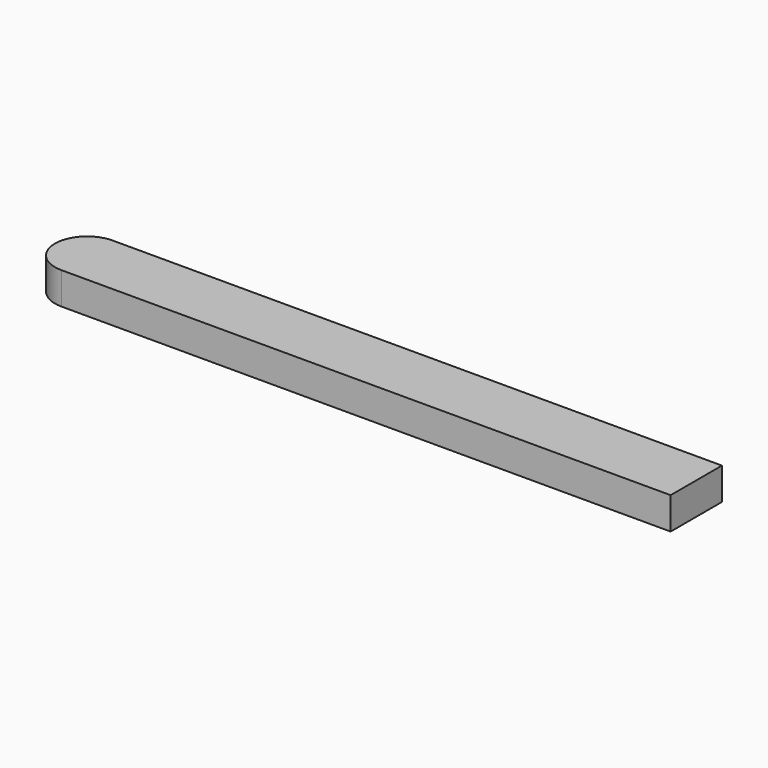
from build123d import *

# Parameters (mm, degrees)
F1_W      = 100
F1_H      = 10
F2_DEPTH  = 5
F3_DEPTH  = 2.5
F4_R      = 5
F5_R      = 4.99999
F6_W      = 3
F6_H      = 0.4
F7_DEPTH  = 0.2
F8_W      = 2.9665668664
F8_H      = 0.4
F9_DEPTH  = 0.2
F10_W     = 2.9665668664
F10_H     = 0.4
F11_DEPTH = 0.2
F12_W     = 2.9335063244
F12_H     = 0.4
F13_DEPTH = 0.2


# Not quite as in the source:
# - a fillet or chamfer is up to 0.001 mm smaller than in the source, because OpenCascade refuses the exact size


with BuildPart() as f2:
    # F1 (on Top) → F2 (new body)
    with BuildSketch(Plane.XY):
        with Locations((32, 0)):
            Rectangle(F1_W, F1_H)
    extrude(amount=F2_DEPTH)

    # F0 (on Top) → F3 (cut)
    with BuildSketch(Plane.XY):
        with BuildLine():
            ThreePointArc((-14.2742941918, -1.9944200271), (-12.7645935136, -1.4660471315), (-12.125, 0))
            ThreePointArc((-12.125, 0), (-12.7645935136, 1.4660471315), (-14.2742941918, 1.9944200271))
            ThreePointArc((-14.2742941918, 1.9944200271), (-16.125, 0), (-14.2742941918, -1.9944200271))
        make_face()
        with BuildLine():
            ThreePointArc((-14.2742941918, 1.9944200271), (-12.7645935136, 1.4660471315), (-12.125, 0))
            ThreePointArc((-12.125, 0), (-12.7645935136, -1.4660471315), (-14.2742941918, -1.9944200271))
            Line((-14.2742941918, -1.9944200271), (-2.1748161696, -2.9001378637))
            ThreePointArc((-2.1748161696, -2.9001378637), (-3.625, 0), (-2.1748161696, 2.9001378637))
            Line((-2.1748161696, 2.9001378637), (-14.2742941918, 1.9944200271))
        make_face()
        with BuildLine():
            Line((0, 3.0629357789), (-2.1748161696, 2.9001378637))
            ThreePointArc((-2.1748161696, 2.9001378637), (-3.625, 0), (-2.1748161696, -2.9001378637))
            Line((-2.1748161696, -2.9001378637), (0, -3.0629357789))
            Line((0, -3.0629357789), (2.1748161696, -2.9001378637))
            ThreePointArc((2.1748161696, -2.9001378637), (3.2422471848, -1.6212520448), (3.625, 0))
            ThreePointArc((3.625, 0), (3.2422471848, 1.6212520448), (2.1748161696, 2.9001378637))
            Line((2.1748161696, 2.9001378637), (0, 3.0629357789))
        make_face()
        with BuildLine():
            ThreePointArc((2.1748161696, 2.9001378637), (0, 3.625), (-2.1748161696, 2.9001378637))
            Line((-2.1748161696, 2.9001378637), (0, 3.0629357789))
            Line((0, 3.0629357789), (2.1748161696, 2.9001378637))
        make_face()
        with BuildLine():
            Line((0, -3.0629357789), (-2.1748161696, -2.9001378637))
            ThreePointArc((-2.1748161696, -2.9001378637), (0, -3.625), (2.1748161696, -2.9001378637))
            Line((2.1748161696, -2.9001378637), (0, -3.0629357789))
        make_face()
        with BuildLine():
            Line((14.2742941918, 1.9944200271), (2.1748161696, 2.9001378637))
            ThreePointArc((2.1748161696, 2.9001378637), (3.2422471848, 1.6212520448), (3.625, 0))
            ThreePointArc((3.625, 0), (3.2422471848, -1.6212520448), (2.1748161696, -2.9001378637))
            Line((2.1748161696, -2.9001378637), (14.2742941918, -1.9944200271))
            ThreePointArc((14.2742941918, -1.9944200271), (12.125, 0), (14.2742941918, 1.9944200271))
        make_face()
        with BuildLine():
            ThreePointArc((16.125, 0), (15.5910471315, 1.3604064864), (14.2742941918, 1.9944200271))
            ThreePointArc((14.2742941918, 1.9944200271), (12.125, 0), (14.2742941918, -1.9944200271))
            ThreePointArc((14.2742941918, -1.9944200271), (15.5910471315, -1.3604064864), (16.125, 0))
        make_face()
    extrude(amount=F3_DEPTH, mode=Mode.SUBTRACT)

    # F4
    f4_edges = [f2.edges().sort_by_distance(p)[0] for p in [
        (-18, 5, 2.5),
    ]]
    fillet(f4_edges, radius=F4_R)

    # F5 (radius 5 in the source; OpenCascade refuses exactly that, so slightly less here)
    f5_edges = [f2.edges().sort_by_distance(p)[0] for p in [
        (-18, -5, 2.5),
    ]]
    fillet(f5_edges, radius=F5_R)

    # F6 (on face) → F7 (join)
    with BuildSketch(Plane(origin=(-0.2280013604, -3.045868522, 0), x_dir=(-0.9972100135, 0.0746470959, 0), z_dir=(0.0746470959, 0.9972100135, 0))):
        with Locations((12.585591441, 0.2)):
            Rectangle(F6_W, F6_H)
        with Locations((3.4522615926, 0.2)):
            Rectangle(F6_W, F6_H)
    extrude(amount=F7_DEPTH)

    # F8 (on face) → F9 (join)
    with BuildSketch(Plane(origin=(0.2280013604, -3.045868522, 0), x_dir=(-0.9972100135, -0.0746470959, 0), z_dir=(-0.0746470959, 0.9972100135, 0))):
        with Locations((-3.4355450259, 0.2)):
            Rectangle(F8_W, F8_H)
        with Locations((-12.6023080078, 0.2)):
            Rectangle(F8_W, F8_H)
    extrude(amount=F9_DEPTH)

    # F10 (on face) → F11 (join)
    with BuildSketch(Plane(origin=(-0.2280013604, 3.045868522, 0), x_dir=(0.9972100135, 0.0746470959, 0), z_dir=(0.0746470959, -0.9972100135, 0))):
        with Locations((-3.4355450259, 0.2)):
            Rectangle(F10_W, F10_H)
        with Locations((-12.6023080078, 0.2)):
            Rectangle(F10_W, F10_H)
    extrude(amount=F11_DEPTH)

    # F12 (on face) → F13 (join)
    with BuildSketch(Plane(origin=(0.2280013604, 3.045868522, 0), x_dir=(0.9972100135, -0.0746470959, 0), z_dir=(-0.0746470959, -0.9972100135, 0))):
        with Locations((12.6188382789, 0.2)):
            Rectangle(F12_W, F12_H)
        with Locations((3.4190147548, 0.2)):
            Rectangle(F12_W, F12_H)
    extrude(amount=F13_DEPTH)


solid = f2.part
